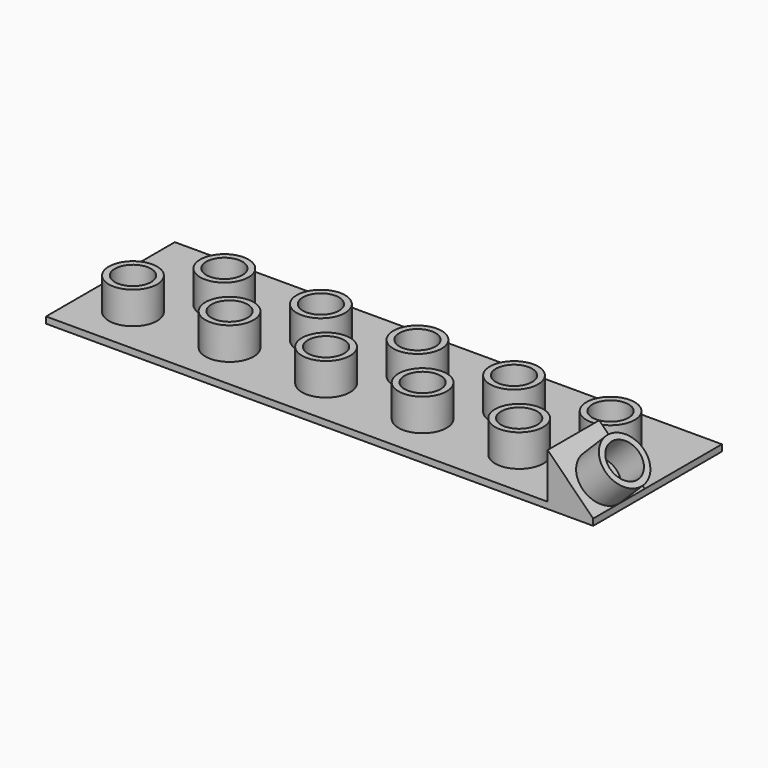
from build123d import *

# Parameters (mm, degrees)
F0_W     = 431.8
F0_H     = 127
F1_DEPTH = 5.08
F2_R     = 19.05
F2_R_2   = 14.2748
F3_DEPTH = 25.4
F5_DEPTH = 50.8
F6_R     = 19.05
F6_R_2   = 14.2875
F7_DEPTH = 25.4


# Not quite as in the source:
# - a feature names something its author has since deleted; it is built from what else it names


with BuildPart() as f1:
    # F0 (on Top) → F1 (new body)
    with BuildSketch(Plane.XY):
        with Locations((215.9, 63.5)):
            Rectangle(F0_W, F0_H)
    extrude(amount=F1_DEPTH)

    # F2 (on face) → F3 (join)
    with BuildSketch(Plane.XY.offset(5.08)):
        with Locations((38.1, 38.1)):
            Circle(F2_R)
        with Locations((38.1, 38.1)):
            Circle(F2_R_2, mode=Mode.SUBTRACT)
        with Locations((76.2, 80.645)):
            Circle(F2_R)
        with Locations((76.2, 80.645)):
            Circle(F2_R_2, mode=Mode.SUBTRACT)
        with Locations((114.3, 38.1)):
            Circle(F2_R)
        with Locations((114.3, 38.1)):
            Circle(F2_R_2, mode=Mode.SUBTRACT)
        with Locations((152.4, 80.645)):
            Circle(F2_R)
        with Locations((152.4, 80.645)):
            Circle(F2_R_2, mode=Mode.SUBTRACT)
        with Locations((190.5, 38.1)):
            Circle(F2_R)
        with Locations((190.5, 38.1)):
            Circle(F2_R_2, mode=Mode.SUBTRACT)
        with Locations((228.6, 80.645)):
            Circle(F2_R)
        with Locations((228.6, 80.645)):
            Circle(F2_R_2, mode=Mode.SUBTRACT)
        with Locations((266.7, 38.1)):
            Circle(F2_R)
        with Locations((266.7, 38.1)):
            Circle(F2_R_2, mode=Mode.SUBTRACT)
        with Locations((304.8, 80.645)):
            Circle(F2_R)
        with Locations((304.8, 80.645)):
            Circle(F2_R_2, mode=Mode.SUBTRACT)
        with Locations((342.9, 38.1)):
            Circle(F2_R)
        with Locations((342.9, 38.1)):
            Circle(F2_R_2, mode=Mode.SUBTRACT)
        with Locations((381, 80.645)):
            Circle(F2_R)
        with Locations((381, 80.645)):
            Circle(F2_R_2, mode=Mode.SUBTRACT)
    extrude(amount=F3_DEPTH)

    # F4 (on face) → F5 (join)
    with BuildSketch(Plane.XZ):
        Polygon((431.8, 5.08), (395.8789755157, 41.0010244843), (395.8789755157, 5.08), align=None)
        Polygon((431.8, 0), (431.8, 5.08), (395.8789755157, 5.08), (0, 5.08), (0, 0), align=None)
    extrude(amount=-F5_DEPTH)

    # F6 (on face) → F7 (join)
    with BuildSketch(Plane(origin=(218.44, 0, 218.44), x_dir=(0.7071067812, 0, -0.7071067812), z_dir=(0.7071067812, 0, 0.7071067812))):
        with Locations((282.6866056679, 25.4)):
            Circle(F6_R)
        with Locations((282.6866056679, 25.4)):
            Circle(F6_R_2, mode=Mode.SUBTRACT)
    extrude(amount=F7_DEPTH)


solid = f1.part
